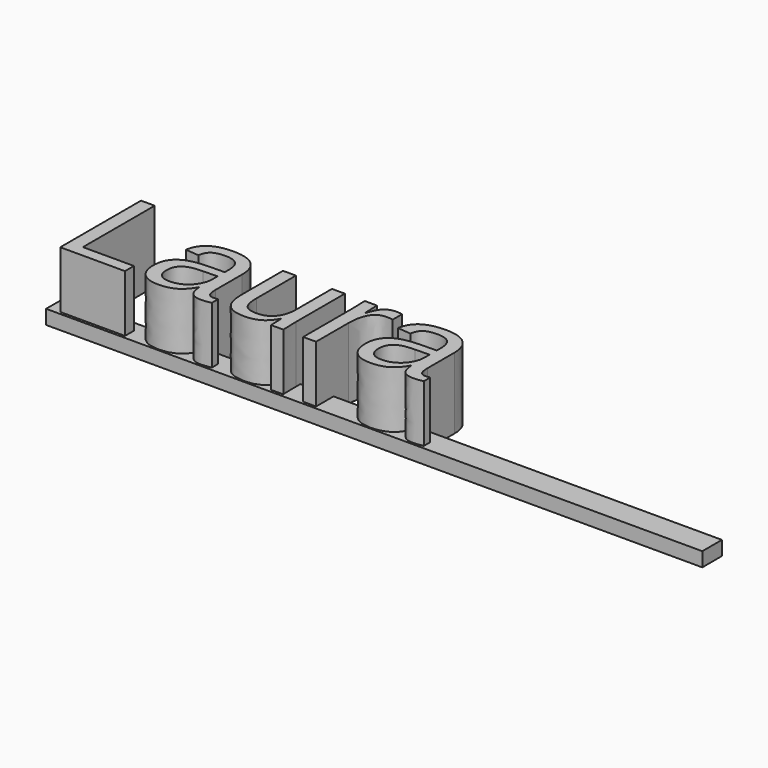
from build123d import *

# Parameters (mm, degrees)
F0_R         = 2
F1_DEPTH     = 4
F2_TEXT_SIZE = 51.4712003577
F4_DEPTH     = 25
F3_W         = 230.2086055279
F3_H         = 8.6075812578
F5_DEPTH     = 5


# Not quite as in the source:
# - Text() gives the source's letters only with a copy of the font that has no kerning and outlines rounded to 1/6400 em; it was checked with that copy


with BuildPart() as f1:
    # F0 (on Top) → F1 (new body)
    with BuildSketch(Plane.XY):
        with Locations((-14.3181821331, 14.8369567469)):
            Circle(F0_R)
    extrude(amount=F1_DEPTH)


with BuildPart() as f4:
    # F2 (on Top) → F4 (new body)
    with BuildSketch(Plane.XY):
        with Locations((0, -44.0219528973)):
            Text('Laura', F2_TEXT_SIZE, font='Arimo', text_align=(TextAlign.LEFT, TextAlign.BOTTOM))
    extrude(amount=F4_DEPTH)


with BuildPart() as f5:
    # F3 (on Top) → F5 (new body)
    with BuildSketch(Plane.XY):
        with Locations((115.1043027639, -40.6633876264)):
            Rectangle(F3_W, F3_H)
    extrude(amount=F5_DEPTH)


solid = Compound([f1.part, f4.part, f5.part])
